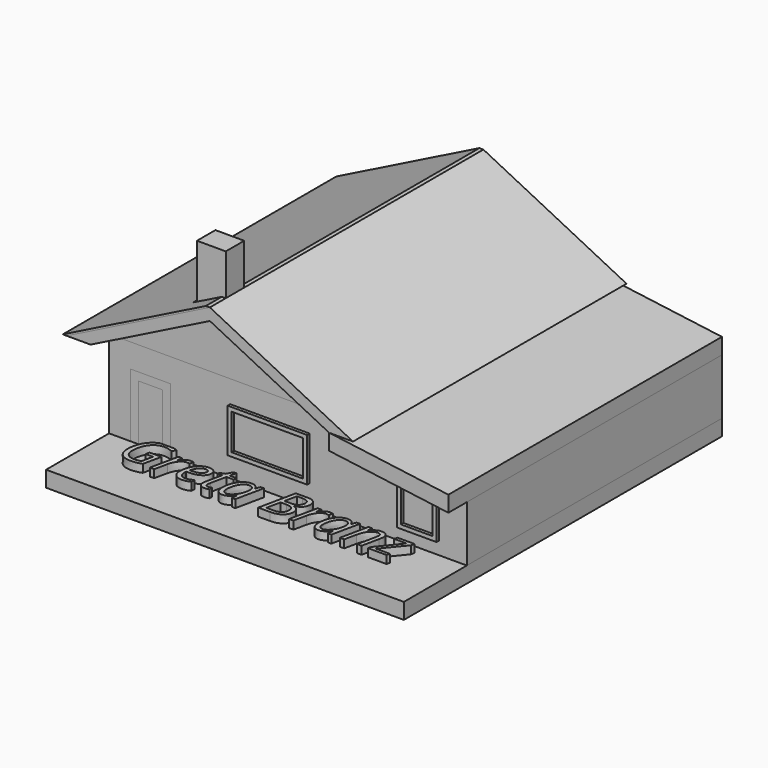
from build123d import *

# Parameters (mm, degrees)
F1_DEPTH      = 914.4
F1_DEPTH_BACK = 12192
F2_DEPTH      = 30.48
F2_DEPTH_BACK = 12192
F3_DEPTH      = 152.4
F3_DEPTH_BACK = 731.52
F0_W          = 4572
F0_H          = 609.6
F4_DEPTH      = 3048
F4_DEPTH_BACK = 12192
F0_W_2        = 3048
F0_H_2        = 1676.4
F0_W_3        = 1524
F0_H_3        = 1524
F0_W_4        = 2743.2
F0_H_4        = 1371.6
F0_W_5        = 1219.2
F0_H_5        = 1219.2
F0_W_6        = 914.4
F0_H_6        = 2133.6
F5_DEPTH      = 30.48
F5_DEPTH_BACK = 12192
F6_DEPTH      = 30.48
F6_DEPTH_BACK = 152.4
F7_DEPTH      = 152.4
F8_W          = 3352.8
F8_H          = 1828.8
F8_W_2        = 3048
F8_H_2        = 1524
F8_W_3        = 2133.6
F8_H_3        = 2133.6
F8_W_4        = 1828.8
F9_DEPTH      = 152.4
F10_TEXT_SIZE = 2024.6182758852
F11_DEPTH     = 304.8


# Not quite as in the source:
# - Text() gives the source's letters only with a copy of the font that has no kerning and outlines rounded to 1/6400 em; it was checked with that copy


with BuildPart() as f1:
    # F0 (on Front) → F1 (new body, two sides)
    with BuildSketch(Plane.XZ) as f1_sk:
        Polygon((-5486.4, 0), (-4572, 0), (0, 2286), (0, 2743.2), (-1104.3480618286, 2191.0259690857), align=None)
        Polygon((0, 2286), (4572, 0), (5486.4, 0), (0, 2743.2), align=None)
    extrude(amount=F1_DEPTH)
    extrude(f1_sk.sketch, amount=-F1_DEPTH_BACK)



with BuildPart() as f1b:
    # F0 (on Front) → F1, piece 2 (new body, two sides)
    with BuildSketch(Plane.XZ) as f1_2_sk:
        Polygon((9144, -603.2345459073), (4572, 0), (4572, -609.6), (9144, -1212.8345459073), align=None)
    extrude(amount=F1_DEPTH)
    extrude(f1_2_sk.sketch, amount=-F1_DEPTH_BACK)


with BuildPart() as f1_1:
    add(f1.part)

    add(f1b.part)  # F2 merges F1b
    # F0 (on Front) → F2 (join, two sides)
    with BuildSketch(Plane.XZ) as f2_sk:
        Polygon((-4572, 0), (0, 0), (0, 2286), align=None)
        Polygon((0, 2286), (0, 0), (4572, 0), align=None)
    extrude(amount=F2_DEPTH)
    extrude(f2_sk.sketch, amount=-F2_DEPTH_BACK)

    # F0 (on Front) → F3 (join, two sides)
    with BuildSketch(Plane.XZ) as f3_sk:
        Polygon((-1104.3480618286, 2191.0259690857), (0, 2743.2), (0, 4324.6259690857), (-1104.3480618286, 4324.6259690857), align=None)
    extrude(amount=F3_DEPTH)
    extrude(f3_sk.sketch, amount=-F3_DEPTH_BACK)


with BuildPart() as f4:
    # F0 (on Front) → F4 (new body, two sides)
    with BuildSketch(Plane.XZ) as f4_sk:
        Polygon((-3743.6601779938, -3352.8), (-4572, -3352.8), (-4572, -3962.4), (4572, -3962.4), (4572, -3352.8), (-2219.6601779938, -3352.8), (-2524.4601779938, -3352.8), (-3438.8601779938, -3352.8), align=None)
        with Locations((6858, -3657.6)):
            Rectangle(F0_W, F0_H)
    extrude(amount=F4_DEPTH)
    extrude(f4_sk.sketch, amount=-F4_DEPTH_BACK)


with BuildPart() as f5:
    # F0 (on Front) → F5 (new body, two sides)
    with BuildSketch(Plane.XZ) as f5_sk:
        Polygon((4572, 0), (0, 0), (-4572, 0), (-4572, -3352.8), (-3743.6601779938, -3352.8), (-3743.6601779938, -914.4), (-2219.6601779938, -914.4), (-2219.6601779938, -3352.8), (4572, -3352.8), (4572, -609.6), align=None)
        with Locations((1595.1515864372, -1696.5094367981)):
            Rectangle(F0_W_2, F0_H_2, mode=Mode.SUBTRACT)
        Polygon((9144, -1212.8345459073), (4572, -609.6), (4572, -3352.8), (9144, -3352.8), align=None)
        with Locations((7319.4003458023, -2096.3345245361)):
            Rectangle(F0_W_3, F0_H_3, mode=Mode.SUBTRACT)
        with Locations((1595.1515864372, -1696.5094367981)):
            Rectangle(F0_W_2, F0_H_2)
        with Locations((1595.1515864372, -1696.5094367981)):
            Rectangle(F0_W_4, F0_H_4, mode=Mode.SUBTRACT)
        with Locations((1595.1515864372, -1696.5094367981)):
            Rectangle(F0_W_4, F0_H_4)
        with Locations((7319.4003458023, -2096.3345245361)):
            Rectangle(F0_W_3, F0_H_3)
        with Locations((7319.4003458023, -2096.3345245361)):
            Rectangle(F0_W_5, F0_H_5, mode=Mode.SUBTRACT)
        with Locations((-2981.6601779938, -2286)):
            Rectangle(F0_W_6, F0_H_6)
        Polygon((-3743.6601779938, -914.4), (-3743.6601779938, -3352.8), (-3438.8601779938, -3352.8), (-3438.8601779938, -1219.2), (-2524.4601779938, -1219.2), (-2524.4601779938, -3352.8), (-2219.6601779938, -3352.8), (-2219.6601779938, -914.4), align=None)
        with Locations((7319.4003458023, -2096.3345245361)):
            Rectangle(F0_W_5, F0_H_5)
    extrude(amount=F5_DEPTH)
    extrude(f5_sk.sketch, amount=-F5_DEPTH_BACK)

    # F0 (on Front) → F7 (join)
    with BuildSketch(Plane.XZ):
        with Locations((1595.1515864372, -1696.5094367981)):
            Rectangle(F0_W_2, F0_H_2)
        with Locations((1595.1515864372, -1696.5094367981)):
            Rectangle(F0_W_4, F0_H_4, mode=Mode.SUBTRACT)
        with Locations((7319.4003458023, -2096.3345245361)):
            Rectangle(F0_W_3, F0_H_3)
        with Locations((7319.4003458023, -2096.3345245361)):
            Rectangle(F0_W_5, F0_H_5, mode=Mode.SUBTRACT)
    extrude(amount=F7_DEPTH)


with BuildPart() as f6:
    # F0 (on Front) → F6 (new body, two sides)
    with BuildSketch(Plane.XZ) as f6_sk:
        Polygon((-3743.6601779938, -914.4), (-3743.6601779938, -3352.8), (-3438.8601779938, -3352.8), (-3438.8601779938, -1219.2), (-2524.4601779938, -1219.2), (-2524.4601779938, -3352.8), (-2219.6601779938, -3352.8), (-2219.6601779938, -914.4), align=None)
    extrude(amount=F6_DEPTH)
    extrude(f6_sk.sketch, amount=-F6_DEPTH_BACK)


with BuildPart() as f9:
    # F8 (on face) + F1_face (on face) → F9 (new body)
    with BuildSketch(Plane(origin=(-4572, 0, 0), x_dir=(0, -1, 0), z_dir=(-1, 0, 0))):
        with Locations((-3779.52, -1828.8)):
            Rectangle(F8_W, F8_H)
        with Locations((-3779.52, -1828.8)):
            Rectangle(F8_W_2, F8_H_2, mode=Mode.SUBTRACT)
        with Locations((-8991.6, -1676.4)):
            Rectangle(F8_W_3, F8_H_3)
        with Locations((-8991.6, -1676.4)):
            Rectangle(F8_W_4, F8_H, mode=Mode.SUBTRACT)
    with BuildSketch(Plane(origin=(-2773.3530755176, 5712.416670892, 1356.5234622412), x_dir=(0, -1, 0), z_dir=(-0.4472135955, 0, 0.894427191))):
        Polygon((6626.816670892, 3100.7030012328), (5864.816670892, 3100.7030012328), (5864.816670892, 1866.0043326983), (4980.896670892, 1866.0043326983), (4980.896670892, 3100.7030012328), (-6479.583329108, 3100.7030012328), (-6479.583329108, -3033.2786746447), (6626.816670892, -3033.2786746447), align=None)
    extrude(amount=F9_DEPTH, dir=(-1, 0, 0))


with BuildPart() as f11:
    # F10 (on face) → F11 (new body)
    with BuildSketch(Plane.XY.offset(-3352.8)):
        with Locations((-3294.5506572723, -1457.7251586374)):
            Text('Greta Branz', F10_TEXT_SIZE, font='Open Sans', font_style=FontStyle.ITALIC, text_align=(TextAlign.LEFT, TextAlign.BOTTOM))
    extrude(amount=F11_DEPTH)


solid = Compound([f1_1.part, f4.part, f5.part, f6.part, f9.part, f11.part])
